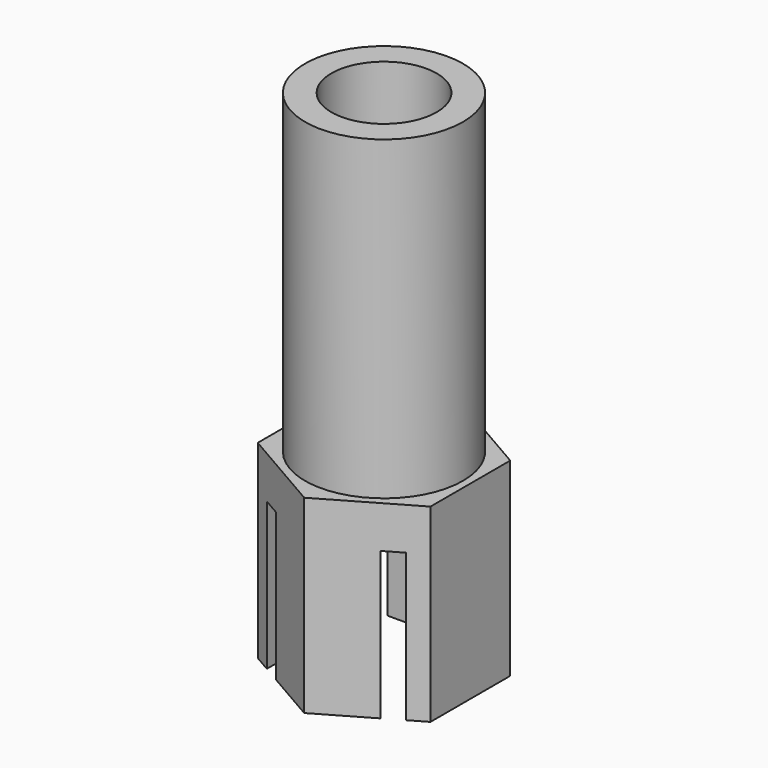
from build123d import *

# Parameters (mm, degrees)
F0_R     = 3.75
F0_R_2   = 2.5
F1_DEPTH = 15
F2_DEPTH = 9
F4_DEPTH = 7


# Not quite as in the source:
# - a feature names something its author has since deleted; it is built from what else it names


with BuildPart() as f1:
    # F0 (on Top) → F1 (new body)
    with BuildSketch(Plane.XY):
        Circle(F0_R)
        Circle(F0_R_2, mode=Mode.SUBTRACT)
    extrude(amount=F1_DEPTH)

    # F0 (on Top) → F2 (join)
    with BuildSketch(Plane.XY):
        Polygon((4.1, -2.3671361037), (4.1, 2.3671361037), (0, 4.7342722074), (-4.1, 2.3671361037), (-4.1, -2.3671361037), (0, -4.7342722074), align=None)
        Circle(F0_R, mode=Mode.SUBTRACT)
        Circle(F0_R)
        Circle(F0_R_2, mode=Mode.SUBTRACT)
        Circle(F0_R_2)
    extrude(amount=-F2_DEPTH)

    # F3 (on face) → F4 (cut)
    with BuildSketch(Plane(origin=(0, 0, -9), x_dir=(1, 0, 0), z_dir=(0, 0, -1))):
        Polygon((-3.3, 2.829016319), (-3.3, 0), (-3.3, -2.829016319), (-2.484232335, -3.3), (0, -3.3), (2.484232335, -3.3), (3.3, -2.829016319), (3.3, 0), (3.3, 2.829016319), (2.484232335, 3.3), (0, 3.3), (-2.484232335, 3.3), align=None)
    extrude(amount=-F4_DEPTH, mode=Mode.SUBTRACT)


solid = f1.part
